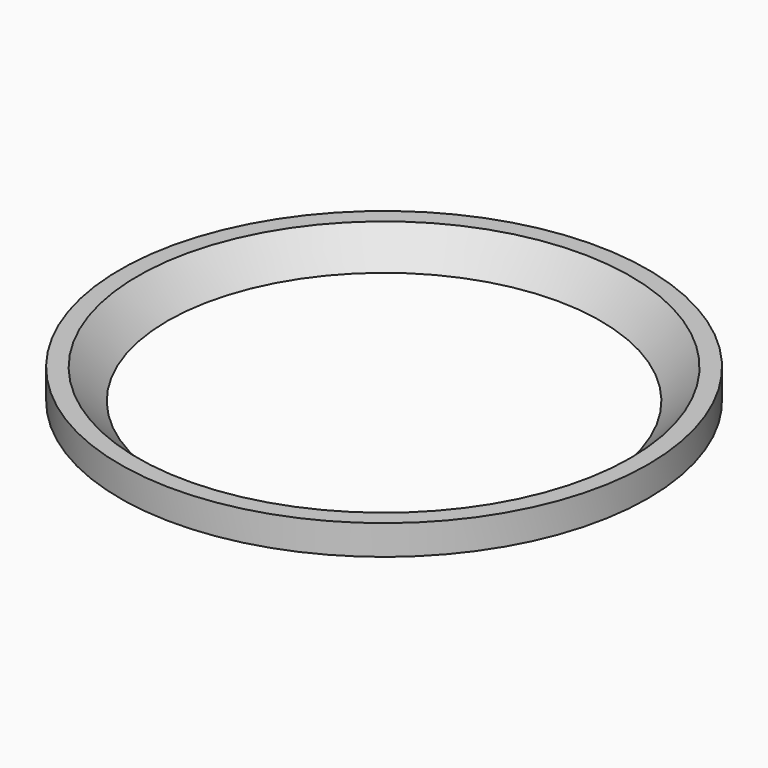
from build123d import *

# Parameters (mm, degrees)
F0_R     = 9.75
F0_R_2   = 8
F1_DEPTH = 1.1
F2_SIZE  = 1.09999


# Not quite as in the source:
# - a fillet or chamfer is up to 0.001 mm smaller than in the source, because OpenCascade refuses the exact size


with BuildPart() as f1:
    # F0 (on Top) → F1 (new body)
    with BuildSketch(Plane.XY):
        Circle(F0_R)
        Circle(F0_R_2, mode=Mode.SUBTRACT)
    extrude(amount=F1_DEPTH)

    # F2 (size 1.1 in the source; OpenCascade refuses exactly that, so slightly less here)
    f2_edges = [f1.edges().sort_by_distance(p)[0] for p in [
        (-8, 0, 1.1),
    ]]
    chamfer(f2_edges, length=F2_SIZE)


solid = f1.part
